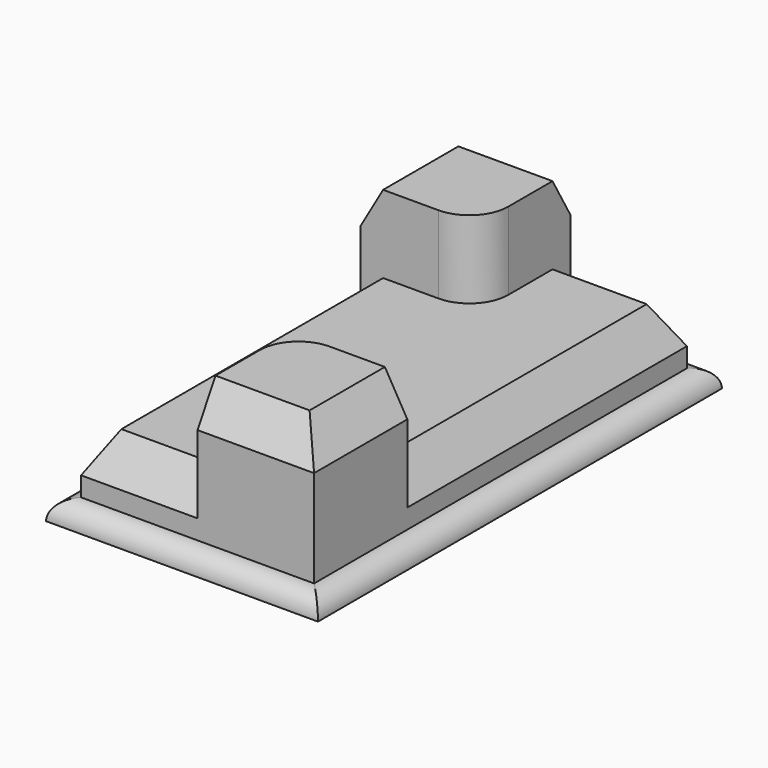
from build123d import *

# Parameters (mm, degrees)
F0_W       = 88.9
F0_H       = 165.1
F1_DEPTH   = 6.35
F2_DEPTH   = 25.4
F3_DEPTH   = 50.8
F4_SIZE2   = 12.7
F4_SIZE    = 7.3323484187
F4_2_SIZE2 = 12.7
F4_2_SIZE  = 7.3323484187
F4_3_SIZE2 = 12.7
F4_3_SIZE  = 7.3323484187
F5_R       = 6.34999


# Not quite as in the source:
# - a fillet or chamfer is up to 0.001 mm smaller than in the source, because OpenCascade refuses the exact size


with BuildPart() as f1:
    # F0 (on Top) → F1 (new body)
    with BuildSketch(Plane.XY):
        with Locations((-5.7064332783, -7.9358178854)):
            Rectangle(F0_W, F0_H)
        Polygon((-43.8064332783, 30.1641821146), (-43.8064332783, 68.2641821146), (-5.7064332783, 68.2641821146), (32.3935667217, 68.2641821146), (32.3935667217, -46.0358178854), (32.3935667217, -84.1358178854), (-5.7064332783, -84.1358178854), (-43.8064332783, -84.1358178854), align=None, mode=Mode.SUBTRACT)
    extrude(amount=F1_DEPTH)

    # F0 (on Top) → F2 (join)
    with BuildSketch(Plane.XY):
        with BuildLine():
            Line((-18.4064332783, 30.1641821146), (-43.8064332783, 30.1641821146))
            Line((-43.8064332783, 30.1641821146), (-43.8064332783, -84.1358178854))
            Line((-43.8064332783, -84.1358178854), (-5.7064332783, -84.1358178854))
            Line((-5.7064332783, -84.1358178854), (-5.7064332783, -58.7358178854))
            ThreePointArc((-5.7064332783, -58.7358178854), (-1.9866893994, -49.7555617643), (6.9935667217, -46.0358178854))
            Line((6.9935667217, -46.0358178854), (32.3935667217, -46.0358178854))
            Line((32.3935667217, -46.0358178854), (32.3935667217, 68.2641821146))
            Line((32.3935667217, 68.2641821146), (-5.7064332783, 68.2641821146))
            Line((-5.7064332783, 68.2641821146), (-5.7064332783, 42.8641821146))
            ThreePointArc((-5.7064332783, 42.8641821146), (-9.4261771573, 33.8839259935), (-18.4064332783, 30.1641821146))
        make_face()
    extrude(amount=F2_DEPTH)

    # F0 (on Top) → F3 (join)
    with BuildSketch(Plane.XY):
        with BuildLine():
            Line((-5.7064332783, 68.2641821146), (-43.8064332783, 68.2641821146))
            Line((-43.8064332783, 68.2641821146), (-43.8064332783, 30.1641821146))
            Line((-43.8064332783, 30.1641821146), (-18.4064332783, 30.1641821146))
            ThreePointArc((-18.4064332783, 30.1641821146), (-9.4261771573, 33.8839259935), (-5.7064332783, 42.8641821146))
            Line((-5.7064332783, 42.8641821146), (-5.7064332783, 68.2641821146))
        make_face()
        with BuildLine():
            Line((-5.7064332783, -58.7358178854), (-5.7064332783, -84.1358178854))
            Line((-5.7064332783, -84.1358178854), (32.3935667217, -84.1358178854))
            Line((32.3935667217, -84.1358178854), (32.3935667217, -46.0358178854))
            Line((32.3935667217, -46.0358178854), (6.9935667217, -46.0358178854))
            ThreePointArc((6.9935667217, -46.0358178854), (-1.9866893994, -49.7555617643), (-5.7064332783, -58.7358178854))
        make_face()
    extrude(amount=F3_DEPTH)

    # F4
    f4_edges = [f1.edges().sort_by_distance(p)[0] for p in [
        (32.393567, 11.114182, 25.4),
        (-43.806433, -26.985818, 25.4),
        (13.343567, 68.264182, 25.4),
        (-24.756433, -84.135818, 25.4),
    ]]
    f4_side = f1.faces().sort_by_distance((-5.706433, -7.935818, 25.4))[0]
    chamfer(f4_edges, length=F4_SIZE, length2=F4_SIZE2, reference=f4_side)

    # F4#2
    f4_2_edges = [f1.edges().sort_by_distance(p)[0] for p in [
        (-24.756433, 68.264182, 50.8),
        (-43.806433, 49.214182, 50.8),
    ]]
    f4_2_side = f1.faces().sort_by_distance((-25.152475, 49.610224, 50.8))[0]
    chamfer(f4_2_edges, length=F4_2_SIZE, length2=F4_2_SIZE2, reference=f4_2_side)

    # F4#3
    f4_3_edges = [f1.edges().sort_by_distance(p)[0] for p in [
        (13.343567, -84.135818, 50.8),
        (32.393567, -65.085818, 50.8),
    ]]
    f4_3_side = f1.faces().sort_by_distance((13.739609, -65.48186, 50.8))[0]
    chamfer(f4_3_edges, length=F4_3_SIZE, length2=F4_3_SIZE2, reference=f4_3_side)

    # F5 (radius 6.35 in the source; OpenCascade refuses exactly that, so slightly less here)
    f5_edges = [f1.edges().sort_by_distance(p)[0] for p in [
        (38.743567, -7.935818, 6.35),
        (-5.706433, 74.614182, 6.35),
        (-50.156433, -7.935818, 6.35),
        (-5.706433, -90.485818, 6.35),
    ]]
    fillet(f5_edges, radius=F5_R)


solid = f1.part
